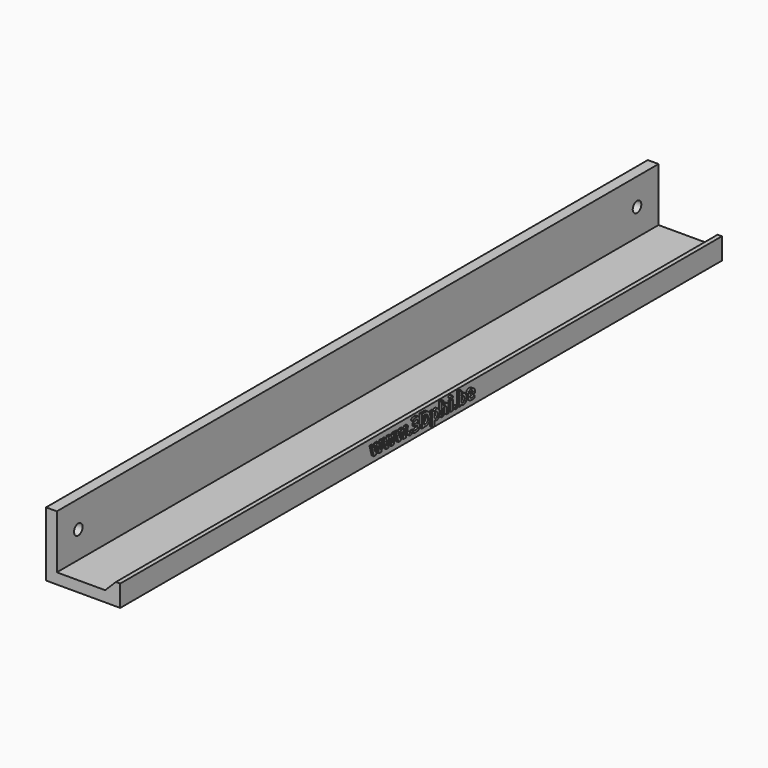
from build123d import *

# Parameters (mm, degrees)
F1_DEPTH     = 350
F2_R         = 2.5
F3_DEPTH     = 25
F4_TEXT_SIZE = 8.3333333333
F5_DEPTH     = 1
F6_SIZE      = 4.99999


# Not quite as in the source:
# - a fillet or chamfer is up to 0.001 mm smaller than in the source, because OpenCascade refuses the exact size
# - Text() gives the source's letters only with a copy of the font that has no kerning and outlines rounded to 1/6400 em; it was checked with that copy


with BuildPart() as f1:
    # F0 (on Front) → F1 (new body)
    with BuildSketch(Plane.XZ):
        Polygon((0, 30), (0, 0), (34.5, 0), (34.5, 10), (32.5, 10), (32.5, 5), (5, 5), (5, 30), align=None)
    extrude(amount=F1_DEPTH)

    # F2 (on face) → F3 (cut)
    with BuildSketch(Plane.YZ.offset(5)):
        with Locations((-337.5, 17.5)):
            Circle(F2_R)
        with Locations((-12.5, 17.5)):
            Circle(F2_R)
    extrude(amount=-F3_DEPTH, mode=Mode.SUBTRACT)

    # F4 (on face) → F5 (join)
    with BuildSketch(Plane.YZ.offset(34.5)):
        with Locations((-205.1041666667, 3)):
            Text('www.3Dphi.be', F4_TEXT_SIZE, font='Open Sans', font_style=FontStyle.BOLD, text_align=(TextAlign.LEFT, TextAlign.BOTTOM))
    extrude(amount=F5_DEPTH)

    # F6 (size 5 in the source; OpenCascade refuses exactly that, so slightly less here)
    f6_edges = [f1.edges().sort_by_distance(p)[0] for p in [
        (32.5, -175, 5),
    ]]
    chamfer(f6_edges, length=F6_SIZE)


solid = f1.part
